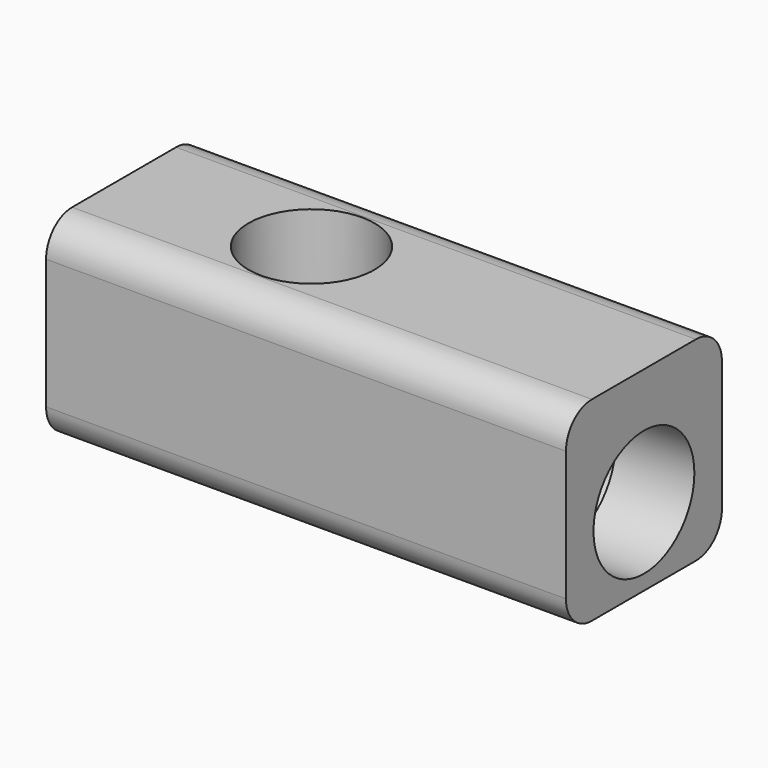
from build123d import *

# Parameters (mm, degrees)
F1_DEPTH = 40
F2_R     = 4.85
F3_DEPTH = 7.07
F4_R     = 4.85
F5_DEPTH = 7.07
F10_SIZE = 1


# Not quite as in the source:
# - a feature names something its author has since deleted; it is built from what else it names


with BuildPart() as f1:
    # F0 (on Right) → F1 (new body)
    with BuildSketch(Plane.YZ):
        with BuildLine():
            ThreePointArc((7.5, 5), (6.767766953, 6.767766953), (5, 7.5))
            Line((5, 7.5), (-5, 7.5))
            ThreePointArc((-5, 7.5), (-6.767766953, 6.767766953), (-7.5, 5))
            Line((-7.5, 5), (-7.5, -5))
            ThreePointArc((-7.5, -5), (-6.767766953, -6.767766953), (-5, -7.5))
            Line((-5, -7.5), (5, -7.5))
            ThreePointArc((5, -7.5), (6.767766953, -6.767766953), (7.5, -5))
            Line((7.5, -5), (7.5, 5))
        make_face()
    extrude(amount=F1_DEPTH)

    # F2 (on face) → F3 (cut)
    with BuildSketch(Plane.YZ.offset(40)):
        with Locations((0, -1.5)):
            Circle(F2_R)
    extrude(amount=-F3_DEPTH, mode=Mode.SUBTRACT)

    # F4 (on face) → F5 (cut)
    with BuildSketch(Plane.YZ):
        with Locations((0, -1.5)):
            Circle(F4_R)
    extrude(amount=F5_DEPTH, mode=Mode.SUBTRACT)

    # F6 (on Front) → F7 (revolve, cut)
    with BuildSketch(Plane.XZ):
        Polygon((32.93, -1.5), (32.93, 1), (10.5341016151, -1), (7.07, 1), (7.07, -1.5), align=None)
    revolve(axis=Axis((20, 0, -1.5), (1, 0, 0)), mode=Mode.SUBTRACT)

    # F8 (on Front) → F9 (revolve, cut)
    with BuildSketch(Plane.XZ):
        Polygon((9.57, 2.1126677044), (11.92, 2.1126677044), (14.42, 2.1126677044), (14.42, 9.1826677044), (9.57, 9.1826677044), align=None)
        Polygon((14.42, 2.1126677044), (11.92, 2.1126677044), (12.92, -0.8873322956), (14.42, -0.7533791963), align=None)
    revolve(axis=Axis((14.42, 0, 2.2679000954), (0, 0, -1)), mode=Mode.SUBTRACT)

    # F10
    f10_edges = [f1.edges().sort_by_distance(p)[0] for p in [
        (32.93, -4.85, -1.5),
        (7.07, -4.85, -1.5),
    ]]
    chamfer(f10_edges, length=F10_SIZE)


solid = f1.part
